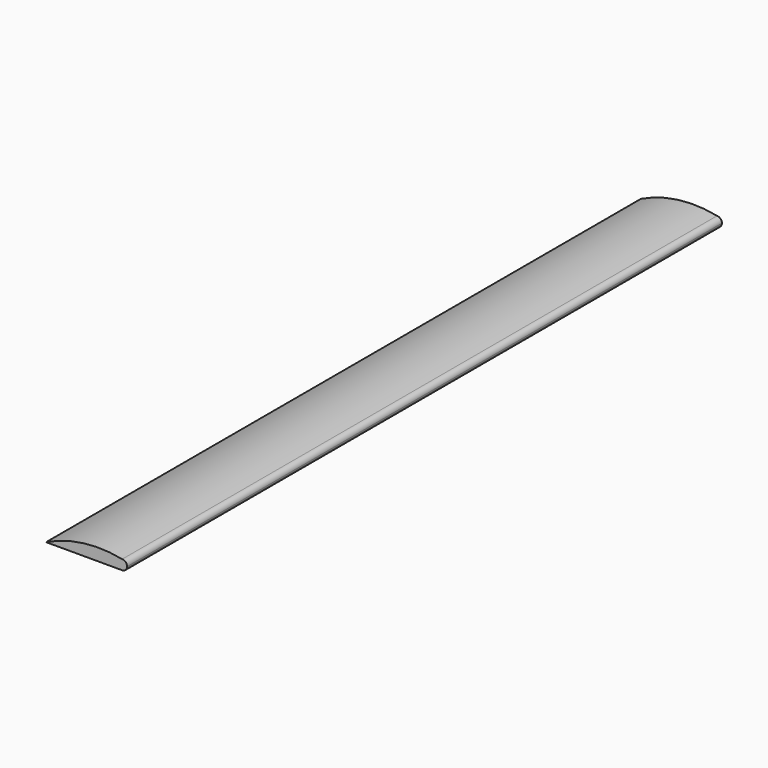
from build123d import *

# Parameters (mm, degrees)
F1_DEPTH = 838.2


with BuildPart() as f1:
    # F0 (on Front) → F1 (new body)
    with BuildSketch(Plane.XZ):
        with BuildLine():
            ThreePointArc((0, -5.5183288966), (3.9020477836, -3.9020477836), (5.5183288966, 0))
            ThreePointArc((5.5183288966, 0), (3.9020477836, 3.9020477836), (0, 5.5183288966))
            ThreePointArc((0, 5.5183288966), (-3.9020477836, 3.9020477836), (-5.5183288966, 0))
            ThreePointArc((-5.5183288966, 0), (-3.9020477836, -3.9020477836), (0, -5.5183288966))
        make_face()
        with BuildLine():
            ThreePointArc((-5.5183288966, 0), (-3.9020477836, 3.9020477836), (0, 5.5183288966))
            ThreePointArc((0, 5.5183288966), (-43.8116245236, 7.1253804433), (-85.7899245391, -5.5183288966))
            Line((-85.7899245391, -5.5183288966), (0, -5.5183288966))
            ThreePointArc((0, -5.5183288966), (-3.9020477836, -3.9020477836), (-5.5183288966, 0))
        make_face()
    extrude(amount=F1_DEPTH)


solid = f1.part
